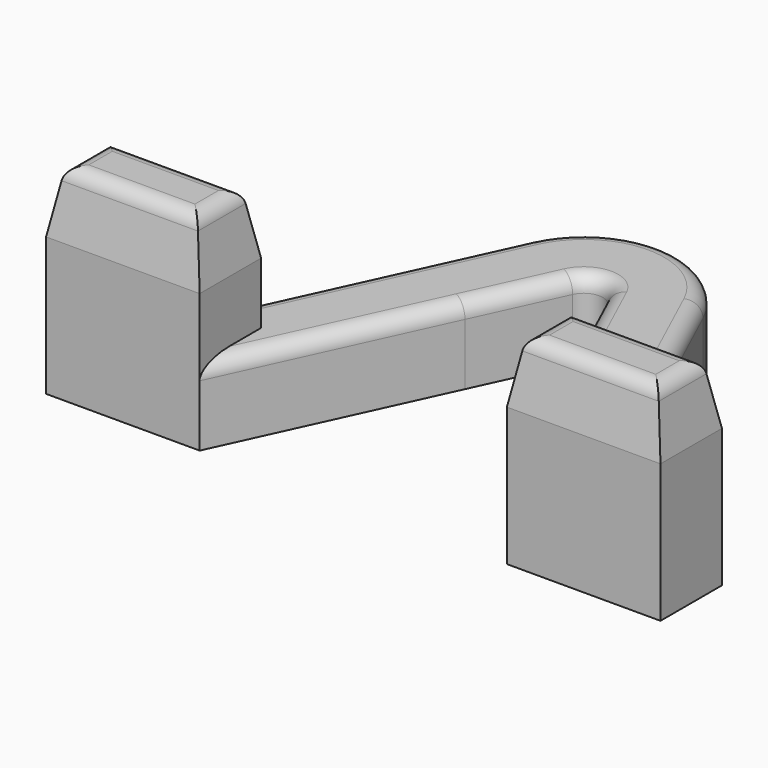
from build123d import *

# Parameters (mm, degrees)
F2_DEPTH  = 6.35
F5_DEPTH  = 5.08
F5_FACE_W = 12.7
F5_FACE_H = 6.35
F6_DEPTH  = 5.08
F6_TAPER  = 10
F7_R      = 1.27


# Not quite as in the source:
# - a variable given as a bare number and used for a length is read in inches; the dataset says mm whatever the document's units were


with BuildPart() as f2:
    # F1 (on Top) → F2 (new body)
    with BuildSketch(Plane.XY):
        Polygon((-25.4, -23.8125), (-12.7, -23.8125), (-12.7, -17.4625), (-16.7687909609, -17.4625), (-25.4, -17.4625), align=None)
        with BuildLine():
            Line((-12.7, -23.8125), (-4.6920856358, -6.4022057634))
            ThreePointArc((-4.6920856358, -6.4022057634), (-7.6835843575, -1.991591743), (-7.2112720666, 3.3168451022))
            Line((-7.2112720666, 3.3168451022), (-16.7687909609, -17.4625))
            Line((-16.7687909609, -17.4625), (-12.7, -17.4625))
            Line((-12.7, -17.4625), (-12.7, -23.8125))
        make_face()
        with BuildLine():
            ThreePointArc((-1.4422544133, 0.6633690204), (0, 1.5875), (1.4422544133, 0.6633690204))
            Line((1.4422544133, 0.6633690204), (4.6920856358, -6.4022057634))
            ThreePointArc((4.6920856358, -6.4022057634), (7.079807059, -3.5889048828), (7.9375, 0))
            ThreePointArc((7.9375, 0), (7.7538177138, 1.6977093717), (7.2112720666, 3.3168451022))
            ThreePointArc((7.2112720666, 3.3168451022), (0, 7.9375), (-7.2112720666, 3.3168451022))
            ThreePointArc((-7.2112720666, 3.3168451022), (-7.6835843575, -1.991591743), (-4.6920856358, -6.4022057634))
            Line((-4.6920856358, -6.4022057634), (-1.4422544133, 0.6633690204))
        make_face()
        with BuildLine():
            ThreePointArc((7.9375, 0), (7.079807059, -3.5889048828), (4.6920856358, -6.4022057634))
            Line((4.6920856358, -6.4022057634), (12.7, -23.8125))
            Line((12.7, -23.8125), (12.7, -17.4625))
            Line((12.7, -17.4625), (16.7687909609, -17.4625))
            Line((16.7687909609, -17.4625), (7.2112720666, 3.3168451022))
            ThreePointArc((7.2112720666, 3.3168451022), (7.7538177138, 1.6977093717), (7.9375, 0))
        make_face()
        Polygon((12.7, -17.4625), (12.7, -23.8125), (25.4, -23.8125), (25.4, -17.4625), (16.7687909609, -17.4625), align=None)
    extrude(amount=F2_DEPTH)

    # F4 (on face) → F5 (join)
    with BuildSketch(Plane.XY.offset(6.35)):
        Polygon((-12.7, -23.8125), (-12.7, -17.4625), (-16.7687909609, -17.4625), (-25.4, -17.4625), (-25.4, -23.8125), align=None)
        Polygon((25.4, -17.4625), (16.7687909609, -17.4625), (12.7, -17.4625), (12.7, -23.8125), (25.4, -23.8125), align=None)
    extrude(amount=F5_DEPTH)

    # F5_face (on face) → F6 (join)
    with BuildSketch(Plane(origin=(19.05, -20.6375, 11.43), x_dir=(1, 0, 0), z_dir=(0, 0, 1))):
        Rectangle(F5_FACE_W, F5_FACE_H)
        with Locations((-38.1, 0)):
            Rectangle(F5_FACE_W, F5_FACE_H)
    extrude(amount=F6_DEPTH, taper=F6_TAPER)

    # F7
    f7_edges = [f2.edges().sort_by_distance(p)[0] for p in [
        (19.05, -18.358241, 16.51),
        (13.595741, -20.6375, 16.51),
        (19.05, -22.916759, 16.51),
        (24.504259, -20.6375, 16.51),
        (-19.05, -18.358241, 16.51),
        (-13.595741, -20.6375, 16.51),
        (-19.05, -22.916759, 16.51),
        (-24.504259, -20.6375, 16.51),
        (7.071127, -11.574565, 6.35),
        (-11.990032, -7.072827, 6.35),
    ]]
    fillet(f7_edges, radius=F7_R)


solid = f2.part
